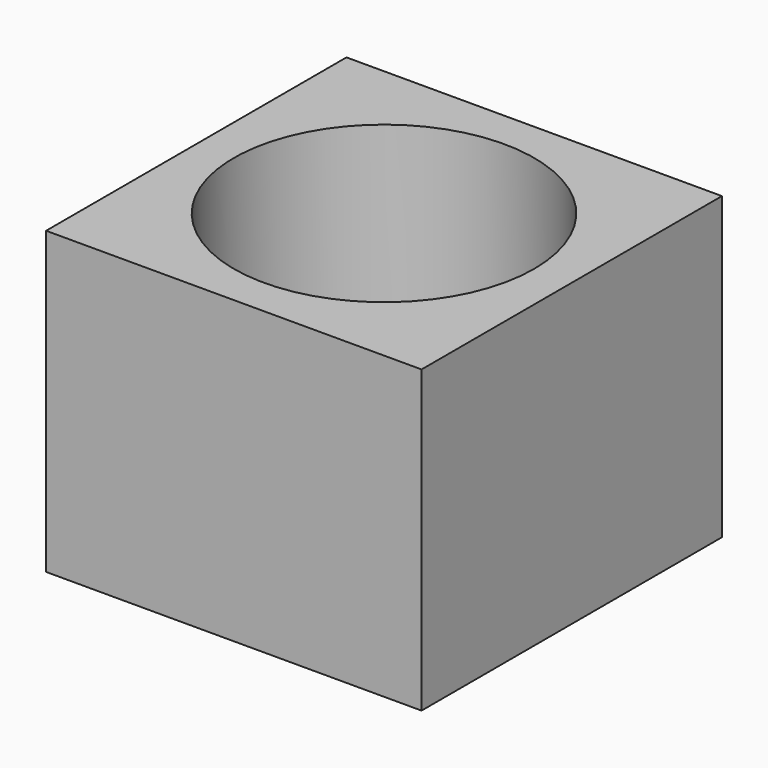
from build123d import *

# Parameters (mm, degrees)
F0_W     = 10
F0_H     = 10
F1_DEPTH = 8
F2_R     = 4
F3_DEPTH = 6
F4_W     = 5.25
F4_H     = 5.25
F5_DEPTH = 3


# Not quite as in the source:
# - a feature names something its author has since deleted; it is built from what else it names


with BuildPart() as f1:
    # F0 (on Top) → F1 (new body)
    with BuildSketch(Plane.XY):
        Rectangle(F0_W, F0_H)
    extrude(amount=F1_DEPTH)

    # F2 (on face) → F3 (cut)
    with BuildSketch(Plane.XY.offset(8)):
        Circle(F2_R)
    extrude(amount=-F3_DEPTH, mode=Mode.SUBTRACT)

    # F4 (on face) → F5 (cut)
    with BuildSketch(Plane.XY):
        Rectangle(F4_W, F4_H)
    extrude(amount=F5_DEPTH, mode=Mode.SUBTRACT)


solid = f1.part
